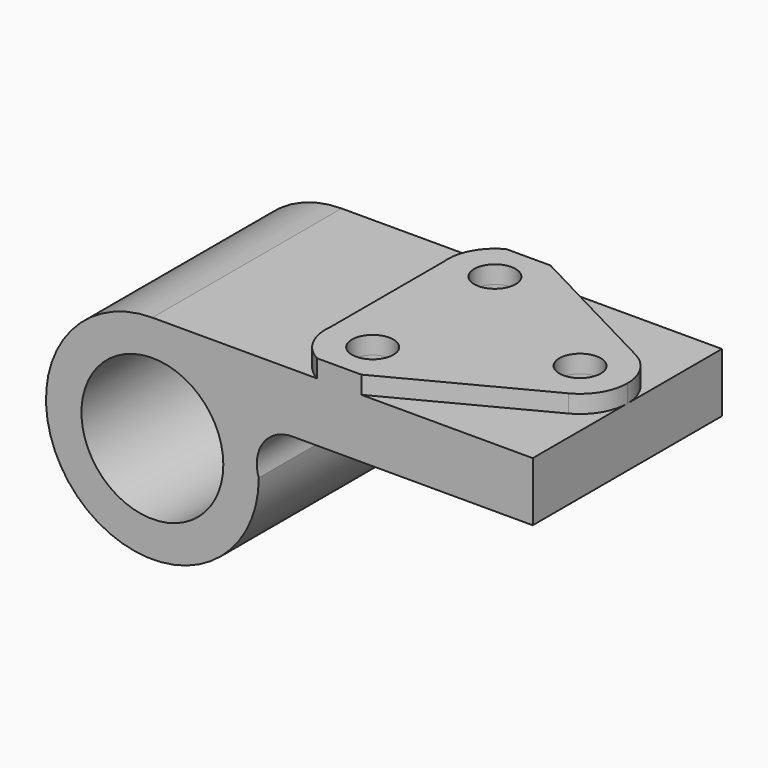
from build123d import *

# Parameters (mm, degrees)
F0_R     = 19.05
F1_DEPTH = 31.75
F3_R     = 5.5626
F4_DEPTH = 4.7752
F5_DEPTH = 57.151


with BuildPart() as f1:
    # F0 (on Front) → F1 (new body, symmetric)
    with BuildSketch(Plane.XZ):
        with BuildLine():
            Line((102.1447438789, 28.575), (0, 28.575))
            ThreePointArc((0, 28.575), (-20.2055762724, -20.2055762724), (28.575, 0))
            ThreePointArc((28.575, 0), (29.7781261877, 8.674261314), (37.5552561211, 12.7))
            Line((37.5552561211, 12.7), (102.1447438789, 12.7))
            Line((102.1447438789, 12.7), (102.1447438789, 28.575))
        make_face()
        Circle(F0_R, mode=Mode.SUBTRACT)
    extrude(amount=F1_DEPTH, both=True)

    # F3 (on face) → F4 (join)
    with BuildSketch(Plane.XY.offset(28.575)):
        with BuildLine():
            ThreePointArc((44.2432574162, 31.75), (38.9330700337, 26.4354220023), (37.5552561211, 19.05))
            Line((37.5552561211, 19.05), (37.5552561211, -19.05))
            ThreePointArc((37.5552561211, -19.05), (38.9330700337, -26.4354220023), (44.2432574161, -31.75))
            Line((44.2432574161, -31.75), (56.097272461, -31.75))
            Line((56.097272461, -31.75), (95.3253515684, -11.2564849399))
            ThreePointArc((95.3253515684, -11.2564849399), (100.3069194614, -6.5805122609), (102.1447438789, -7.87e-08))
            ThreePointArc((102.1447438789, -7.87e-08), (100.3069195022, 6.5805121935), (95.3253515684, 11.2564849399))
            Line((95.3253515684, 11.2564849399), (56.097272461, 31.75))
            Line((56.097272461, 31.75), (44.2432574162, 31.75))
        make_face()
        with Locations((50.170148764, -20.5178159314)):
            Circle(F3_R, mode=Mode.SUBTRACT)
        with Locations((50.170148764, 20.5178159314)):
            Circle(F3_R, mode=Mode.SUBTRACT)
        with Locations((89.4447438789, 0)):
            Circle(F3_R, mode=Mode.SUBTRACT)
    extrude(amount=F4_DEPTH)

    # F5 (cut, through all): faces of the model
    f5_faces = [f1.faces().sort_by_distance(p)[0] for p in [
        (89.4447438789, 0, 28.575),
        (50.170148764, -20.5178159314, 28.575),
        (50.170148764, 20.5178159314, 28.575),
    ]]
    extrude(f5_faces, amount=-F5_DEPTH, mode=Mode.SUBTRACT)


solid = f1.part
